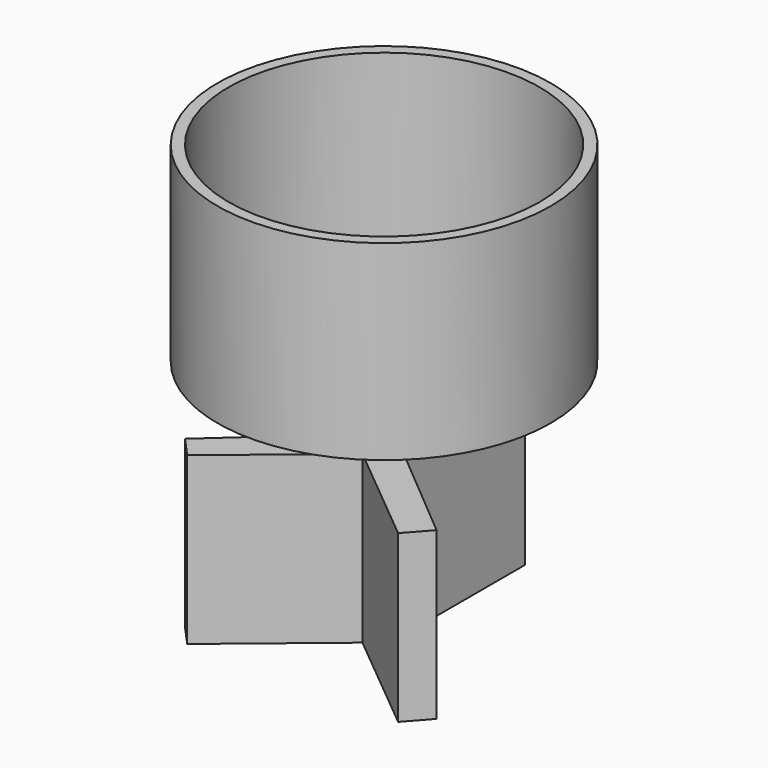
from build123d import *
from build123d import SkipClean  # not in build123d's __all__

# Parameters (mm, degrees)
F0_R     = 37.5
F1_DEPTH = 3
F2_R     = 37.5
F2_R_2   = 35
F3_DEPTH = 40
F5_DEPTH = 56.2
F6_DEPTH = 18.8


with BuildPart() as f1:
    # F0 (on Top) → F1 (new body)
    with BuildSketch(Plane.XY):
        Circle(F0_R)
    extrude(amount=F1_DEPTH)

    # F2 (on face) → F3 (join)
    with BuildSketch(Plane.XY.offset(3)):
        Circle(F2_R)
        Circle(F2_R_2, mode=Mode.SUBTRACT)
    extrude(amount=F3_DEPTH)

    # F4 (on face) → F5 (join)
    with BuildSketch(Plane.XY.offset(3)):
        Polygon((3.8241918664, 34.7904520892), (-4.540327032, 34.7042566617), (-4.540327032, 5.5238307981), (-4.540327032, 0), (-27.9463561921, -21.0713354011), (-23.733683415, -25.7237686111), (0, -6.0903779231), (23.733683415, -25.7237686111), (28.2858054869, -20.6134230043), (3.8241918664, 0), align=None)
    extrude(amount=-F5_DEPTH)

    # F4 (on face) → F6 (cut)
    with BuildSketch(Plane.XY.offset(3)):
        with BuildLine():
            ThreePointArc((23.733683415, -25.7237686111), (26.1349519697, -23.2801264073), (28.2858054869, -20.6134230043))
            Line((28.2858054869, -20.6134230043), (23.733683415, -25.7237686111))
        make_face()
        Polygon((3.8241918664, 34.7904520892), (-4.540327032, 34.7042566617), (-4.540327032, 5.5238307981), (-4.540327032, 0), (-27.9463561921, -21.0713354011), (-23.733683415, -25.7237686111), (0, -6.0903779231), (23.733683415, -25.7237686111), (28.2858054869, -20.6134230043), (3.8241918664, 0), align=None)
    with SkipClean():  # cleaning this boolean's faces spoils the solid; the shape is the same uncleaned
        extrude(amount=-F6_DEPTH, mode=Mode.SUBTRACT)


solid = f1.part
